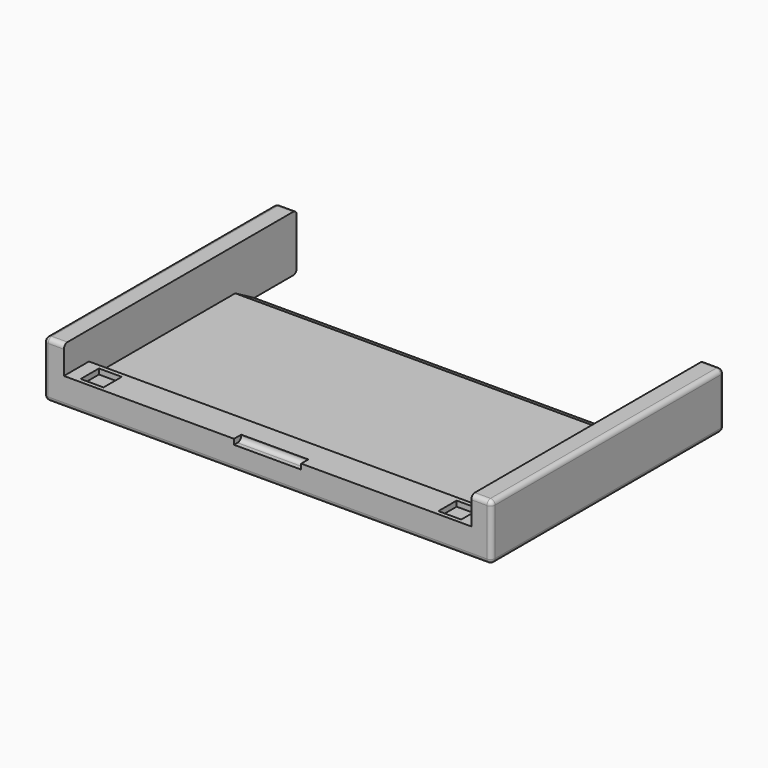
from build123d import *

# Parameters (mm, degrees)
F0_W     = 65
F0_H     = 12.5
F1_DEPTH = 50
F3_DEPTH = 45.5
F4_W     = 5.1
F4_H     = 5.1
F5_DEPTH = 1.2
F6_R     = 1
F7_W     = 15
F7_H     = 1.1837528777
F8_DEPTH = 2
F9_R     = 1


# Not quite as in the source:
# - a pattern or mirror of a feature is missing from the dataset's text; its kind, count and spacing are read off the source's solid


with BuildPart() as f1:
    # F0 (on Right) → F1 (new body, symmetric)
    with BuildSketch(Plane.YZ):
        Rectangle(F0_W, F0_H)
    extrude(amount=F1_DEPTH, both=True)

    # F2 (on Right) → F3 (cut, symmetric)
    with BuildSketch(Plane.YZ):
        Polygon((-32.5, 6.25), (-32.5, 0), (-25.5, 0), (-25.5, -3.1976206858), (15.3335404618, -3.1976206858), (20.620416518, -6.25), (32.5, -6.25), (32.5, 6.25), align=None)
    extrude(amount=F3_DEPTH, both=True, mode=Mode.SUBTRACT)

    # F4 (on face) → F5 (cut)
    with BuildSketch(Plane.XY):
        with Locations((-39.95, -29.0152)):
            Rectangle(F4_W, F4_H)
    f5 = extrude(amount=-F5_DEPTH, mode=Mode.SUBTRACT)

    # F5_copies: F5 across plane
    add(f5.mirror(Plane(origin=(0, 0, 0), x_dir=(0, 0, 1), z_dir=(1, 0, 0))), mode=Mode.SUBTRACT)

    # F6
    f6_edges = [f1.edges().sort_by_distance(p)[0] for p in [
        (-47.75, -32.5, 6.25),
        (47.75, -32.5, 6.25),
        (-50, 0, 6.25),
        (-47.75, 32.5, 6.25),
        (47.75, 32.5, 6.25),
        (50, 0, 6.25),
        (-50, -32.5, 0),
        (50, -32.5, 0),
        (0, -32.5, -6.25),
        (50, 0, -6.25),
        (50, 32.5, 0),
        (-50, 0, -6.25),
        (-50, 32.5, 0),
        (-47.75, 32.5, -6.25),
        (47.75, 32.5, -6.25),
    ]]
    fillet(f6_edges, radius=F6_R)

    # F7 (on face) → F8 (cut)
    with BuildSketch(Plane.XZ.offset(32.5)):
        with Locations((0, -0.5918764388)):
            Rectangle(F7_W, F7_H)
    extrude(amount=-F8_DEPTH, mode=Mode.SUBTRACT)

    # F9
    f9_edges = [f1.edges().sort_by_distance(p)[0] for p in [
        (0, -30.5, -1.183753),
    ]]
    fillet(f9_edges, radius=F9_R)


solid = f1.part
